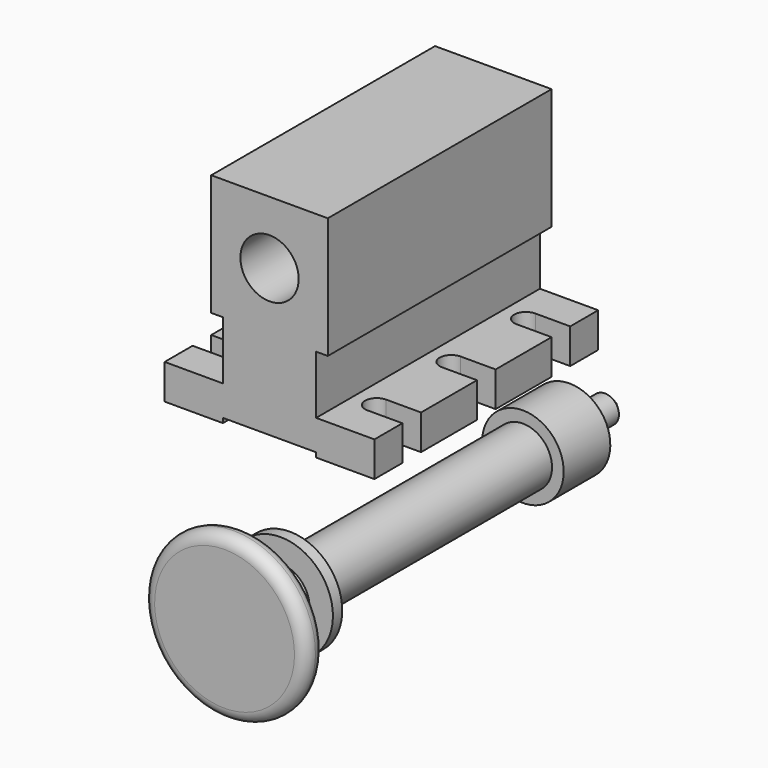
from build123d import *

# Parameters (mm, degrees)
F0_R     = 12.5
F1_DEPTH = 60
F3_DEPTH = 25
F6_R     = 4.99999


# Not quite as in the source:
# - a fillet or chamfer is up to 0.001 mm smaller than in the source, because OpenCascade refuses the exact size


with BuildPart() as f1:
    # F0 (on Front) → F1 (new body, symmetric)
    with BuildSketch(Plane.XZ):
        Polygon((-20, 2), (0, 2), (20, 2), (20, 0), (45, 0), (45, 15), (20, 15), (20, 40), (25, 40), (25, 92), (-25, 92), (-25, 40), (-20, 40), (-20, 15), (-45, 15), (-45, 0), (-20, 0), align=None)
        with Locations((0, 65)):
            Circle(F0_R, mode=Mode.SUBTRACT)
    extrude(amount=F1_DEPTH, both=True)

    # F2 (on face) → F3 (cut)
    with BuildSketch(Plane(origin=(0, 0, 0), x_dir=(1, 0, 0), z_dir=(0, 0, -1))):
        with BuildLine():
            ThreePointArc((-30, 35), (-25, 40), (-30, 45))
            Line((-30, 45), (-50, 45))
            ThreePointArc((-50, 45), (-55, 40), (-50, 35))
            Line((-50, 35), (-30, 35))
        make_face()
        with BuildLine():
            ThreePointArc((-30, -5), (-25, 0), (-30, 5))
            Line((-30, 5), (-50, 5))
            ThreePointArc((-50, 5), (-55, 0), (-50, -5))
            Line((-50, -5), (-30, -5))
        make_face()
        with BuildLine():
            ThreePointArc((-30, -45), (-25, -40), (-30, -35))
            Line((-30, -35), (-50, -35))
            ThreePointArc((-50, -35), (-55, -40), (-50, -45))
            Line((-50, -45), (-30, -45))
        make_face()
        with BuildLine():
            Line((50, 45), (30, 45))
            ThreePointArc((30, 45), (25, 40), (30, 35))
            Line((30, 35), (50, 35))
            ThreePointArc((50, 35), (55, 40), (50, 45))
        make_face()
        with BuildLine():
            Line((50, 5), (30, 5))
            ThreePointArc((30, 5), (25, 0), (30, -5))
            Line((30, -5), (50, -5))
            ThreePointArc((50, -5), (55, 0), (50, 5))
        make_face()
        with BuildLine():
            Line((50, -35), (30, -35))
            ThreePointArc((30, -35), (25, -40), (30, -45))
            Line((30, -45), (50, -45))
            ThreePointArc((50, -45), (55, -40), (50, -35))
        make_face()
    extrude(amount=-F3_DEPTH, mode=Mode.SUBTRACT)


with BuildPart() as f5:
    # F4 (on Right) → F5 (revolve)
    with BuildSketch(Plane.YZ):
        Polygon((-84.121281445, -61.381906271), (125.878718555, -61.381906271), (119.878718555, -55.381906271), (100.878718555, -55.381906271), (100.878718555, -43.881906271), (75.878718555, -43.881906271), (75.878718555, -48.881906271), (-49.121281445, -48.881906271), (-49.121281445, -38.881906271), (-54.121281445, -38.881906271), (-54.121281445, -48.881906271), (-74.121281445, -48.881906271), (-74.121281445, -26.381906271), (-84.121281445, -26.381906271), align=None)
    revolve(axis=Axis((0, 20.878718555, -61.381906271), (0, -1, 0)))

    # F6 (radius 5 in the source; OpenCascade refuses exactly that, so slightly less here)
    f6_edges = [f5.edges().sort_by_distance(p)[0] for p in [
        (0, -74.121281, -96.381906),
        (0, -84.121281, -96.381906),
    ]]
    fillet(f6_edges, radius=F6_R)


solid = Compound([f1.part, f5.part])
